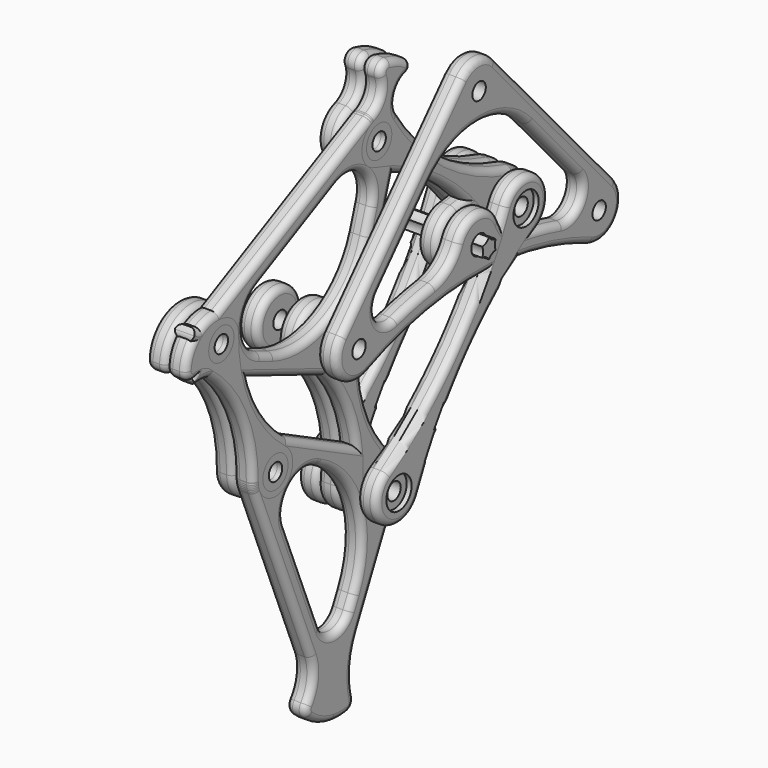
from build123d import *

# Parameters (mm, degrees)
F9_START        = -20
F4_R            = 14.25
F4_R_2          = 4.25
F9_DEPTH        = 10
F10_DEPTH       = 25
F5_R            = 4.25
F11_DEPTH       = 10
F12_DEPTH       = 10
F6_R            = 4.25
F13_DEPTH       = 10
F14_START       = -10
F7_R            = 4.25
F14_DEPTH       = 10
F15_START       = 10
F8_R            = 4.25
F15_DEPTH       = 10
F16_F1_R        = 3.3333333333
F16_F2_R        = 3.3333333333
F16_2_T1_DEPTH  = 111.6
F16_2_T3_DEPTH  = 23.6921609305
F16_2_T5_DEPTH  = 83
F16_2_T7_DEPTH  = 9.0519604966
F16_2_T9_DEPTH  = 55.2336790395
F16_2_T11_DEPTH = 12.4143797947
F16_2_T13_DEPTH = 80.2
F16_2_T16_ANGLE = 132.0850519137
F16_2_T18_ANGLE = 201.4453377433
F16_2_T20_ANGLE = 201.4453377433
F16_2_T22_ANGLE = 100.7027482307
F16_2_T24_ANGLE = 100.7027482307
F16_2_T26_ANGLE = 54.6379434109
F16_2_T28_ANGLE = 54.6379434109
F16_2_T30_ANGLE = 134.1832559662
F16_2_T32_ANGLE = 134.1832559662
F16_2_T34_ANGLE = 93.7316921202
F16_2_T36_ANGLE = 134.1832559662
F16_2_T38_ANGLE = 134.1832559662
F16_2_T40_ANGLE = 93.7316921202
F16_2_T42_ANGLE = 132.0850519137
F16_2_T44_ANGLE = 93.7316921202
F16_2_T46_ANGLE = 93.7316921202
F16_3_F1_R      = 3.3333333333
F16_4_F1_R      = 3.3333333333
F16_4_F2_R      = 3.3333333333
F16_4_F3_R      = 3.3333333333
F16_4_F4_R      = 3.3333333333
F16_5_F1_R      = 3.3333333333
F16_5_F2_R      = 3.3333333333
F16_6_F1_R      = 3.3333333333
F16_7_F1_R      = 3.3333333333
F16_8_F1_R      = 3.3333333333
F16_8_F2_R      = 3.3333333333
F16_9_F1_R      = 3.3333333333
F16_9_F2_R      = 3.3333333333
F17_R           = 8
F17_R_2         = 4.25
F18_DEPTH       = 2.5
F19_R           = 8
F19_R_2         = 4.25
F20_DEPTH       = 2.5
F21_R           = 8
F21_R_2         = 4.25
F22_DEPTH       = 2.5
F23_R           = 8
F23_R_2         = 4.25
F24_DEPTH       = 2.5


# Not quite as in the source:
# - a fillet or chamfer that OpenCascade refuses, or shapes differently, is made with other operations: its cross-section is extruded or revolved along the edge and cut away or added


with BuildPart() as f9:
    # F4 (on Right) → F9 (new body)
    with BuildSketch(Plane.YZ.offset(F9_START)):
        with Locations((-76, -15.6)):
            Circle(F4_R)
        with Locations((-76, -15.6)):
            Circle(F4_R_2, mode=Mode.SUBTRACT)
    extrude(amount=-F9_DEPTH)

    # F16: fillet of radius 3.3333333333 on 3 edges, made by hand

    # F16_f1
    f16_f1_edges = [f9.edges().sort_by_distance(p)[0] for p in [
        (-20, -90.25, -15.6),
    ]]
    fillet(f16_f1_edges, radius=F16_F1_R)

    # F16_f2
    f16_f2_edges = [f9.edges().sort_by_distance(p)[0] for p in [
        (-30, -90.25, -15.6),
    ]]
    fillet(f16_f2_edges, radius=F16_F2_R)


with BuildPart() as f10:
    # F3 (on Right) → F10 (new body, symmetric)
    with BuildSketch(Plane.YZ):
        with BuildLine():
            ThreePointArc((-4.2835398746, 2.4731028997), (-3.6961524227, 0), (-4.2835398746, -2.4731028997))
            ThreePointArc((-4.2835398746, -2.4731028997), (-1.8480762114, -3.2009618943), (0, -4.9462057994))
            ThreePointArc((0, -4.9462057994), (1.8480762114, -3.2009618943), (4.2835398746, -2.4731028997))
            ThreePointArc((4.2835398746, -2.4731028997), (3.6961524227, 0), (4.2835398746, 2.4731028997))
            ThreePointArc((4.2835398746, 2.4731028997), (1.8480762114, 3.2009618943), (0, 4.9462057994))
            ThreePointArc((0, 4.9462057994), (-1.8480762114, 3.2009618943), (-4.2835398746, 2.4731028997))
        make_face()
    extrude(amount=F10_DEPTH, both=True)


with BuildPart() as f11:
    # F5 (on Right) → F11 (new body)
    with BuildSketch(Plane.YZ):
        with BuildLine():
            Line((-57.1063179985, 76.2227923438), (-157.0028723597, 26.471024267))
            ThreePointArc((-157.0028723597, 26.471024267), (-162.7660308401, 21.2166273966), (-164.900160038, 13.7154158472))
            ThreePointArc((-164.900160038, 13.7154158472), (-162.4248725051, 5.6892931022), (-155.8589465196, 0.4515158405))
            Line((-155.8589465196, 0.4515158405), (-81.2087864816, -28.8639000068))
            ThreePointArc((-81.2087864816, -28.8639000068), (-69.8818983437, -28.469783686), (-62.4252123986, -19.9344713145))
            Line((-62.4252123986, -19.9344713145), (-37.1788180755, 59.1327126096))
            ThreePointArc((-37.1788180755, 59.1327126096), (-41.4768983317, 74.2840781563), (-57.1063179985, 76.2227923438))
        make_face()
        with Locations((-76, -15.6)):
            Circle(F5_R, mode=Mode.SUBTRACT)
        with Locations((-150.650160038, 13.7154158472)):
            Circle(F5_R, mode=Mode.SUBTRACT)
        with BuildLine():
            ThreePointArc((-125.7090220308, -0.6450333714), (-136.4139116441, 14.3413005541), (-127.0655051666, 30.2092608039))
            Line((-127.0655051666, 30.2092608039), (-77.6241591027, 54.8326764813))
            ThreePointArc((-77.6241591027, 54.8326764813), (-60.030313022, 52.6502896918), (-55.192016778, 35.5945832725))
            Line((-55.192016778, 35.5945832725), (-58.9681412066, 23.7684380854))
            ThreePointArc((-58.9681412066, 23.7684380854), (-82.1181016563, -2.730216314), (-117.2834571963, -3.9537863164))
            Line((-117.2834571963, -3.9537863164), (-125.7090220308, -0.6450333714))
        make_face(mode=Mode.SUBTRACT)
        with Locations((-50.7536056769, 63.4671839241)):
            Circle(F5_R, mode=Mode.SUBTRACT)
        with BuildLine():
            ThreePointArc((-164.900160038, 13.7154158472), (-162.7660308401, 21.2166273966), (-157.0028723597, 26.471024267))
            ThreePointArc((-157.0028723597, 26.471024267), (-161.4609160942, 25.4223284212), (-165.9189598286, 26.471024267))
            ThreePointArc((-165.9189598286, 26.471024267), (-167.5662735959, 24.188567011), (-168.8749908257, 21.6964769273))
            ThreePointArc((-168.8749908257, 21.6964769273), (-165.9488558838, 18.1734595817), (-164.900160038, 13.7154158472))
        make_face()
        with BuildLine():
            ThreePointArc((-155.8589465196, 0.4515158405), (-162.4248725051, 5.6892931022), (-164.900160038, 13.7154158472))
            ThreePointArc((-164.900160038, 13.7154158472), (-165.9488558838, 9.2573721128), (-168.8749908257, 5.7343547672))
            ThreePointArc((-168.8749908257, 5.7343547672), (-167.7693516826, 3.5776118128), (-166.4096773207, 1.5713058254))
            ThreePointArc((-166.4096773207, 1.5713058254), (-161.0587017415, 1.7238146329), (-155.8589465196, 0.4515158405))
        make_face()
    extrude(amount=F11_DEPTH)

    # F16#2: fillet of radius 3.3333333333 on 28 edges, made by hand

    # F16_2_s2 → F16_2_t1 (cut)
    with BuildSketch(Plane(origin=(0, -15.3399823815, -7.6398155134), x_dir=(1, 0, 0), z_dir=(0, -0.8951304154, -0.4458043734))):
        with BuildLine():
            ThreePointArc((3.3333333333, 93.6875860907), (0.9763107294, 92.7112753613), (0, 90.3542527573))
            Line((0, 90.3542527573), (0, 93.6875860907))
            Line((0, 93.6875860907), (3.3333333333, 93.6875860907))
        make_face()
        with BuildLine():
            ThreePointArc((6.6666666667, 93.6875860907), (9.0236892706, 92.7112753613), (10, 90.3542527573))
            Line((10, 90.3542527573), (10, 93.6875860907))
            Line((10, 93.6875860907), (6.6666666667, 93.6875860907))
        make_face()
    extrude(amount=F16_2_T1_DEPTH, mode=Mode.SUBTRACT)

    # F16_2_s4 → F16_2_t3 (cut)
    with BuildSketch(Plane.YZ.offset(-6.8460804653)):
        with BuildLine():
            ThreePointArc((-167.6064610002, 24.1233767851), (-168.0886966243, 22.1185143512), (-167.2992446495, 20.2135759911))
            ThreePointArc((-167.2992446495, 20.2135759911), (-168.0468911695, 20.9977716348), (-168.8749908257, 21.6964769273))
            ThreePointArc((-168.8749908257, 21.6964769273), (-168.2825299449, 22.9317776388), (-167.6064610002, 24.1233767851))
        make_face()
        with BuildLine():
            ThreePointArc((-167.2992446495, 7.2172557033), (-168.0886966243, 5.3123173433), (-167.6064610002, 3.3074549094))
            ThreePointArc((-167.6064610002, 3.3074549094), (-168.2825299449, 4.4990540557), (-168.8749908257, 5.7343547672))
            ThreePointArc((-168.8749908257, 5.7343547672), (-168.0468911695, 6.4330600597), (-167.2992446495, 7.2172557033))
        make_face()
    extrude(amount=F16_2_T3_DEPTH, mode=Mode.SUBTRACT)

    # F16_2_s6 → F16_2_t5 (cut)
    with BuildSketch(Plane(origin=(0, -11.5518984951, -36.1784764705), x_dir=(1, 0, 0), z_dir=(0, 0.3041734256, 0.9526166738))):
        with BuildLine():
            ThreePointArc((3.3333333333, -53.4037617685), (0.9763107294, -54.3800724979), (0, -56.7370951019))
            Line((0, -56.7370951019), (0, -53.4037617685))
            Line((0, -53.4037617685), (3.3333333333, -53.4037617685))
        make_face()
        with BuildLine():
            ThreePointArc((6.6666666667, -53.4037617685), (9.0236892706, -54.3800724979), (10, -56.7370951019))
            Line((10, -56.7370951019), (10, -53.4037617685))
            Line((10, -53.4037617685), (6.6666666667, -53.4037617685))
        make_face()
    extrude(amount=F16_2_T5_DEPTH, mode=Mode.SUBTRACT)

    # F16_2_s8 → F16_2_t7 (cut)
    with BuildSketch(Plane(origin=(0, -100.2678414461, 39.3755816009), x_dir=(1, 0, 0), z_dir=(0, -0.9308000005, 0.3655288759))):
        with BuildLine():
            ThreePointArc((3.3333333333, -46.5506745758), (0.9763107294, -47.5269853052), (0, -49.8840079092))
            Line((0, -49.8840079092), (0, -46.5506745758))
            Line((0, -46.5506745758), (3.3333333333, -46.5506745758))
        make_face()
        with BuildLine():
            ThreePointArc((6.6666666667, -46.5506745758), (9.0236892706, -47.5269853052), (10, -49.8840079092))
            Line((10, -49.8840079092), (10, -46.5506745758))
            Line((10, -46.5506745758), (6.6666666667, -46.5506745758))
        make_face()
    extrude(amount=F16_2_T7_DEPTH, mode=Mode.SUBTRACT)

    # F16_2_s10 → F16_2_t9 (cut)
    with BuildSketch(Plane(origin=(0, -89.7572132841, -44.7020428992), x_dir=(1, 0, 0), z_dir=(0, 0.8951304154, 0.4458043734))):
        with BuildLine():
            ThreePointArc((3.3333333333, -83.6875860907), (0.9763107294, -84.66389682), (0, -87.020919424))
            Line((0, -87.020919424), (0, -83.6875860907))
            Line((0, -83.6875860907), (3.3333333333, -83.6875860907))
        make_face()
        with BuildLine():
            ThreePointArc((6.6666666667, -83.6875860907), (9.0236892706, -84.66389682), (10, -87.020919424))
            Line((10, -87.020919424), (10, -83.6875860907))
            Line((10, -83.6875860907), (6.6666666667, -83.6875860907))
        make_face()
    extrude(amount=F16_2_T9_DEPTH, mode=Mode.SUBTRACT)

    # F16_2_s12 → F16_2_t11 (cut)
    with BuildSketch(Plane(origin=(0, 5.2074638633, 16.3088438607), x_dir=(1, 0, 0), z_dir=(0, -0.3041734256, -0.9526166738))):
        with BuildLine():
            ThreePointArc((3.3333333333, 63.4037617685), (0.9763107294, 62.4274510392), (0, 60.0704284352))
            Line((0, 60.0704284352), (0, 63.4037617685))
            Line((0, 63.4037617685), (3.3333333333, 63.4037617685))
        make_face()
        with BuildLine():
            ThreePointArc((6.6666666667, 63.4037617685), (9.0236892706, 62.4274510392), (10, 60.0704284352))
            Line((10, 60.0704284352), (10, 63.4037617685))
            Line((10, 63.4037617685), (6.6666666667, 63.4037617685))
        make_face()
    extrude(amount=F16_2_T11_DEPTH, mode=Mode.SUBTRACT)

    # F16_2_s14 → F16_2_t13 (cut)
    with BuildSketch(Plane(origin=(0, -135.1880420105, 53.0888837625), x_dir=(1, 0, 0), z_dir=(0, 0.9308000005, -0.3655288759))):
        with BuildLine():
            ThreePointArc((6.6666666667, 56.5506745758), (9.0236892706, 55.5743638465), (10, 53.2173412425))
            Line((10, 53.2173412425), (10, 56.5506745758))
            Line((10, 56.5506745758), (6.6666666667, 56.5506745758))
        make_face()
        with BuildLine():
            ThreePointArc((3.3333333333, 56.5506745758), (0.9763107294, 55.5743638465), (0, 53.2173412425))
            Line((0, 53.2173412425), (0, 56.5506745758))
            Line((0, 56.5506745758), (3.3333333333, 56.5506745758))
        make_face()
    extrude(amount=F16_2_T13_DEPTH, mode=Mode.SUBTRACT)

    # F16_2_s15 → F16_2_t16 (revolve, cut)
    with BuildSketch(Plane(origin=(0, -108.6934062806, 42.6843345459), x_dir=(1, 0, 0), z_dir=(0, 0.9308000005, -0.3655288759))):
        with BuildLine():
            ThreePointArc((6.6666666667, 46.5506745758), (9.0236892706, 47.5269853052), (10, 49.8840079092))
            Line((10, 49.8840079092), (10, 46.5506745758))
            Line((10, 46.5506745758), (6.6666666667, 46.5506745758))
        make_face()
    revolve(axis=Axis((10, -119.5323707365, 15.0834833251), (-1, 0, 0)), revolution_arc=F16_2_T16_ANGLE, mode=Mode.SUBTRACT)

    # F16_2_s17 → F16_2_t18 (revolve, cut)
    with BuildSketch(Plane(origin=(0, -166.3384411937, -31.4981407109), x_dir=(1, 0, 0), z_dir=(0, -0.9825392613, -0.1860553681))):
        with BuildLine():
            ThreePointArc((3.3333333333, 56.0170482127), (0.9763107294, 56.9933589421), (0, 59.350381546))
            Line((0, 59.350381546), (0, 56.0170482127))
            Line((0, 56.0170482127), (3.3333333333, 56.0170482127))
        make_face()
    revolve(axis=Axis((0, -174.900160038, 13.7154158472), (-1, 0, 0)), revolution_arc=F16_2_T18_ANGLE, mode=Mode.SUBTRACT)

    # F16_2_s19 → F16_2_t20 (revolve, cut)
    with BuildSketch(Plane(origin=(0, -166.3384411937, -31.4981407109), x_dir=(1, 0, 0), z_dir=(0, -0.9825392613, -0.1860553681))):
        with BuildLine():
            ThreePointArc((6.6666666667, 56.0170482127), (9.0236892706, 56.9933589421), (10, 59.350381546))
            Line((10, 59.350381546), (10, 56.0170482127))
            Line((10, 56.0170482127), (6.6666666667, 56.0170482127))
        make_face()
    revolve(axis=Axis((10, -174.900160038, 13.7154158472), (-1, 0, 0)), revolution_arc=F16_2_T20_ANGLE, mode=Mode.SUBTRACT)

    # F16_2_s21 → F16_2_t22 (revolve, cut)
    with BuildSketch(Plane(origin=(0, -115.2365367426, -57.3915835903), x_dir=(1, 0, 0), z_dir=(0, 0.8951304154, 0.4458043734))):
        with BuildLine():
            ThreePointArc((3.3333333333, -93.6875860907), (0.9763107294, -92.7112753613), (0, -90.3542527573))
            Line((0, -90.3542527573), (0, -93.6875860907))
            Line((0, -93.6875860907), (3.3333333333, -93.6875860907))
        make_face()
    revolve(axis=Axis((0, -161.4609160942, 35.4223284212), (-1, 0, 0)), revolution_arc=F16_2_T22_ANGLE, mode=Mode.SUBTRACT)

    # F16_2_s23 → F16_2_t24 (revolve, cut)
    with BuildSketch(Plane(origin=(0, -115.2365367426, -57.3915835903), x_dir=(1, 0, 0), z_dir=(0, 0.8951304154, 0.4458043734))):
        with BuildLine():
            ThreePointArc((6.6666666667, -93.6875860907), (9.0236892706, -92.7112753613), (10, -90.3542527573))
            Line((10, -90.3542527573), (10, -93.6875860907))
            Line((10, -93.6875860907), (6.6666666667, -93.6875860907))
        make_face()
    revolve(axis=Axis((10, -161.4609160942, 35.4223284212), (-1, 0, 0)), revolution_arc=F16_2_T24_ANGLE, mode=Mode.SUBTRACT)

    # F16_2_s25 → F16_2_t26 (revolve, cut)
    with BuildSketch(Plane(origin=(0, -122.5752098671, -80.2042759428), x_dir=(1, 0, 0), z_dir=(0, -0.8367852502, -0.5475312274))):
        with BuildLine():
            ThreePointArc((3.3333333333, 94.1406373476), (0.9763107294, 95.116948077), (0, 97.4739706809))
            Line((0, 97.4739706809), (0, 94.1406373476))
            Line((0, 94.1406373476), (3.3333333333, 94.1406373476))
        make_face()
    revolve(axis=Axis((0, -163.1695240376, -18.164484169), (-1, 0, 0)), revolution_arc=F16_2_T26_ANGLE, mode=Mode.SUBTRACT)

    # F16_2_s27 → F16_2_t28 (revolve, cut)
    with BuildSketch(Plane(origin=(0, -122.5752098671, -80.2042759428), x_dir=(1, 0, 0), z_dir=(0, -0.8367852502, -0.5475312274))):
        with BuildLine():
            ThreePointArc((6.6666666667, 94.1406373476), (9.0236892706, 95.116948077), (10, 97.4739706809))
            Line((10, 97.4739706809), (10, 94.1406373476))
            Line((10, 94.1406373476), (6.6666666667, 94.1406373476))
        make_face()
    revolve(axis=Axis((10, -163.1695240376, -18.164484169), (-1, 0, 0)), revolution_arc=F16_2_T28_ANGLE, mode=Mode.SUBTRACT)

    # F16_2_s29 → F16_2_t30 (revolve, cut)
    with BuildSketch(Plane(origin=(0, 13.694495828, 42.8887074536), x_dir=(1, 0, 0), z_dir=(0, -0.3041734256, -0.9526166738))):
        with BuildLine():
            ThreePointArc((3.3333333333, 53.4037617685), (0.9763107294, 54.3800724979), (0, 56.7370951019))
            Line((0, 56.7370951019), (0, 53.4037617685))
            Line((0, 53.4037617685), (3.3333333333, 53.4037617685))
        make_face()
    revolve(axis=Axis((0, -50.7536056769, 63.4671839241), (1, 0, 0)), revolution_arc=F16_2_T30_ANGLE, mode=Mode.SUBTRACT)

    # F16_2_s31 → F16_2_t32 (revolve, cut)
    with BuildSketch(Plane(origin=(0, 13.694495828, 42.8887074536), x_dir=(1, 0, 0), z_dir=(0, -0.3041734256, -0.9526166738))):
        with BuildLine():
            ThreePointArc((6.6666666667, 53.4037617685), (9.0236892706, 54.3800724979), (10, 56.7370951019))
            Line((10, 56.7370951019), (10, 53.4037617685))
            Line((10, 53.4037617685), (6.6666666667, 53.4037617685))
        make_face()
    revolve(axis=Axis((10, -50.7536056769, 63.4671839241), (1, 0, 0)), revolution_arc=F16_2_T32_ANGLE, mode=Mode.SUBTRACT)

    # F16_2_s33 → F16_2_t34 (revolve, cut)
    with BuildSketch(Plane(origin=(0, 1.4313394348, 4.4826986736), x_dir=(1, 0, 0), z_dir=(0, 0.3041734256, 0.9526166738))):
        with BuildLine():
            ThreePointArc((3.3333333333, -63.4037617685), (0.9763107294, -62.4274510392), (0, -60.0704284352))
            Line((0, -60.0704284352), (0, -63.4037617685))
            Line((0, -63.4037617685), (3.3333333333, -63.4037617685))
        make_face()
    revolve(axis=Axis((0, -101.1123053029, 37.2251989359), (-1, 0, 0)), revolution_arc=F16_2_T34_ANGLE, mode=Mode.SUBTRACT)

    # F16_2_s35 → F16_2_t36 (revolve, cut)
    with BuildSketch(Plane(origin=(0, -40.3158672201, -20.0786272217), x_dir=(1, 0, 0), z_dir=(0, -0.8951304154, -0.4458043734))):
        with BuildLine():
            ThreePointArc((3.3333333333, 83.6875860907), (0.9763107294, 84.66389682), (0, 87.020919424))
            Line((0, 87.020919424), (0, 83.6875860907))
            Line((0, 83.6875860907), (3.3333333333, 83.6875860907))
        make_face()
    revolve(axis=Axis((0, -70.4729887352, 40.4738444846), (-1, 0, 0)), revolution_arc=F16_2_T36_ANGLE, mode=Mode.SUBTRACT)

    # F16_2_s37 → F16_2_t38 (revolve, cut)
    with BuildSketch(Plane(origin=(0, -40.3158672201, -20.0786272217), x_dir=(1, 0, 0), z_dir=(0, -0.8951304154, -0.4458043734))):
        with BuildLine():
            ThreePointArc((6.6666666667, 83.6875860907), (9.0236892706, 84.66389682), (10, 87.020919424))
            Line((10, 87.020919424), (10, 83.6875860907))
            Line((10, 83.6875860907), (6.6666666667, 83.6875860907))
        make_face()
    revolve(axis=Axis((10, -70.4729887352, 40.4738444846), (-1, 0, 0)), revolution_arc=F16_2_T38_ANGLE, mode=Mode.SUBTRACT)

    # F16_2_s39 → F16_2_t40 (revolve, cut)
    with BuildSketch(Plane(origin=(0, 1.4313394348, 4.4826986736), x_dir=(1, 0, 0), z_dir=(0, 0.3041734256, 0.9526166738))):
        with BuildLine():
            ThreePointArc((6.6666666667, -63.4037617685), (9.0236892706, -62.4274510392), (10, -60.0704284352))
            Line((10, -60.0704284352), (10, -63.4037617685))
            Line((10, -63.4037617685), (6.6666666667, -63.4037617685))
        make_face()
    revolve(axis=Axis((10, -101.1123053029, 37.2251989359), (-1, 0, 0)), revolution_arc=F16_2_T40_ANGLE, mode=Mode.SUBTRACT)

    # F16_2_s41 → F16_2_t42 (revolve, cut)
    with BuildSketch(Plane(origin=(0, -108.6934062806, 42.6843345459), x_dir=(1, 0, 0), z_dir=(0, 0.9308000005, -0.3655288759))):
        with BuildLine():
            ThreePointArc((3.3333333333, 46.5506745758), (0.9763107294, 47.5269853052), (0, 49.8840079092))
            Line((0, 49.8840079092), (0, 46.5506745758))
            Line((0, 46.5506745758), (3.3333333333, 46.5506745758))
        make_face()
    revolve(axis=Axis((0, -119.5323707365, 15.0834833251), (-1, 0, 0)), revolution_arc=F16_2_T42_ANGLE, mode=Mode.SUBTRACT)

    # F16_2_s43 → F16_2_t44 (revolve, cut)
    with BuildSketch(Plane(origin=(0, -60.5378819724, 23.7734679153), x_dir=(1, 0, 0), z_dir=(0, -0.9308000005, 0.3655288759))):
        with BuildLine():
            ThreePointArc((6.6666666667, -56.5506745758), (9.0236892706, -55.5743638465), (10, -53.2173412425))
            Line((10, -53.2173412425), (10, -56.5506745758))
            Line((10, -56.5506745758), (6.6666666667, -56.5506745758))
        make_face()
    revolve(axis=Axis((10, -76, -15.6), (1, 0, 0)), revolution_arc=F16_2_T44_ANGLE, mode=Mode.SUBTRACT)

    # F16_2_s45 → F16_2_t46 (revolve, cut)
    with BuildSketch(Plane(origin=(0, -60.5378819724, 23.7734679153), x_dir=(1, 0, 0), z_dir=(0, -0.9308000005, 0.3655288759))):
        with BuildLine():
            ThreePointArc((3.3333333333, -56.5506745758), (0.9763107294, -55.5743638465), (0, -53.2173412425))
            Line((0, -53.2173412425), (0, -56.5506745758))
            Line((0, -56.5506745758), (3.3333333333, -56.5506745758))
        make_face()
    revolve(axis=Axis((0, -76, -15.6), (1, 0, 0)), revolution_arc=F16_2_T46_ANGLE, mode=Mode.SUBTRACT)


with BuildPart() as f11b:
    # F5 (on Right) → F11, piece 2 (new body)
    with BuildSketch(Plane.YZ):
        with BuildLine():
            ThreePointArc((-110.0171751391, -44.4920792731), (-126.0763947693, -46.799791208), (-129.5669264658, -62.6440412054))
            Line((-129.5669264658, -62.6440412054), (-93.817508921, -149.9170955083))
            Line((-93.817508921, -149.9170955083), (-80.052473801, -183.5209061437))
            Line((-80.052473801, -183.5209061437), (-63.817508921, -149.9170955083))
            Line((-63.817508921, -149.9170955083), (-37.8736864923, -96.2174846691))
            ThreePointArc((-37.8736864923, -96.2174846691), (-37.218611188, -85.4153913463), (-44.3415008039, -77.2680735467))
            Line((-44.3415008039, -77.2680735467), (-110.0171751391, -44.4920792731))
        make_face()
        with BuildLine():
            ThreePointArc((-69.5436558742, -138.7818275874), (-78.8542275315, -144.4269408432), (-87.8015966731, -138.2222141207))
            Line((-87.8015966731, -138.2222141207), (-110.1854942304, -83.5776564974))
            ThreePointArc((-110.1854942304, -83.5776564974), (-106.6843293072, -67.6851400706), (-90.5761883844, -65.3703981397))
            Line((-90.5761883844, -65.3703981397), (-89.1351981073, -66.0895363829))
            ThreePointArc((-89.1351981073, -66.0895363829), (-64.1907642182, -94.6215284794), (-66.4848447814, -132.4505722079))
            Line((-66.4848447814, -132.4505722079), (-69.5436558742, -138.7818275874))
        make_face(mode=Mode.SUBTRACT)
        with Locations((-116.3803620382, -57.2424656393)):
            Circle(F5_R, mode=Mode.SUBTRACT)
        with Locations((-50.7046877031, -90.0184599129)):
            Circle(F5_R, mode=Mode.SUBTRACT)
        with BuildLine():
            Line((-80.052473801, -183.5209061437), (-93.817508921, -149.9170955083))
            ThreePointArc((-93.817508921, -149.9170955083), (-92.4766246704, -159.9565618129), (-96.2262873625, -169.3655407133))
            ThreePointArc((-96.2262873625, -169.3655407133), (-97.1781166541, -172.8165666329), (-95.5788811028, -176.0193786083))
            ThreePointArc((-95.5788811028, -176.0193786083), (-88.3662640694, -180.9097278853), (-80.052473801, -183.5209061437))
        make_face()
        with BuildLine():
            Line((-63.817508921, -149.9170955083), (-80.052473801, -183.5209061437))
            ThreePointArc((-80.052473801, -183.5209061437), (-75.315298055, -183.8972810119), (-70.5781223089, -183.5209061437))
            ThreePointArc((-70.5781223089, -183.5209061437), (-67.1842215616, -181.3220496315), (-66.5268751351, -177.331883229))
            ThreePointArc((-66.5268751351, -177.331883229), (-67.6067408069, -163.3838862214), (-63.817508921, -149.9170955083))
        make_face()
    extrude(amount=F11_DEPTH)

    # F16#4: fillet of radius 3.3333333333 on 31 edges, made by hand

    # F16_4_f1
    f16_4_f1_edges = [f11b.edges().sort_by_distance(p)[0] for p in [
        (0, -37.218611188, -85.4153913463),
        (0, -77.1793379715, -60.8800764099),
        (0, -126.0763947693, -46.799791208),
        (0, -111.6922176934, -106.2805683569),
        (0, -92.4766246704, -159.9565618129),
        (0, -97.1781166541, -172.8165666329),
        (0, -83.9371052765, -182.6316583365),
        (0, -67.1842215616, -181.3220496315),
        (0, -67.6067408069, -163.3838862214),
        (0, -50.8455977066, -123.0672900887),
    ]]
    fillet(f16_4_f1_edges, radius=F16_4_F1_R)

    # F16_4_f2
    f16_4_f2_edges = [f11b.edges().sort_by_distance(p)[0] for p in [
        (10, -37.218611188, -85.4153913463),
        (10, -77.1793379715, -60.8800764099),
        (10, -126.0763947693, -46.799791208),
        (10, -111.6922176934, -106.2805683569),
        (10, -92.4766246704, -159.9565618129),
        (10, -97.1781166541, -172.8165666329),
        (10, -83.9371052765, -182.6316583365),
        (10, -67.1842215616, -181.3220496315),
        (10, -67.6067408069, -163.3838862214),
        (10, -50.8455977066, -123.0672900887),
    ]]
    fillet(f16_4_f2_edges, radius=F16_4_F2_R)

    # F16_4_f3
    f16_4_f3_edges = [f11b.edges().sort_by_distance(p)[0] for p in [
        (0, -78.8542275315, -144.4269408432),
        (0, -98.9935454517, -110.899935309),
        (0, -106.6843293072, -67.6851400706),
        (0, -89.8556932459, -65.7299672613),
        (0, -64.1907642182, -94.6215284794),
        (0, -68.0142503278, -135.6161998976),
    ]]
    fillet(f16_4_f3_edges, radius=F16_4_F3_R)

    # F16_4_f4
    f16_4_f4_edges = [f11b.edges().sort_by_distance(p)[0] for p in [
        (10, -78.8542275315, -144.4269408432),
        (10, -98.9935454517, -110.899935309),
        (10, -106.6843293072, -67.6851400706),
        (10, -89.8556932459, -65.7299672613),
        (10, -64.1907642182, -94.6215284794),
        (10, -68.0142503278, -135.6161998976),
    ]]
    fillet(f16_4_f4_edges, radius=F16_4_F4_R)


with BuildPart() as f12:
    # F5 (on Right) → F12 (new body)
    with BuildSketch(Plane.YZ):
        with BuildLine():
            Line((27.7700369033, 18.2177811599), (-1.9482561751, 14.1161892123))
            ThreePointArc((-1.9482561751, 14.1161892123), (-14.1161892123, -1.9482561751), (1.9482561751, -14.1161892123))
            Line((1.9482561751, -14.1161892123), (31.6665492535, -10.0145972646))
            ThreePointArc((31.6665492535, -10.0145972646), (43.8344822907, 6.0498481227), (27.7700369033, 18.2177811599))
        make_face()
        with BuildLine():
            ThreePointArc((-5.1961524227, -3), (-4.1961524227, 0), (-5.1961524227, 3))
            ThreePointArc((-5.1961524227, 3), (-2.0980762114, 3.6339745962), (0, 6))
            ThreePointArc((0, 6), (2.0980762114, 3.6339745962), (5.1961524227, 3))
            ThreePointArc((5.1961524227, 3), (4.1961524227, 0), (5.1961524227, -3))
            ThreePointArc((5.1961524227, -3), (2.0980762114, -3.6339745962), (0, -6))
            ThreePointArc((0, -6), (-2.0980762114, -3.6339745962), (-5.1961524227, -3))
        make_face(mode=Mode.SUBTRACT)
        with Locations((29.7182930784, 4.1015919476)):
            Circle(F5_R, mode=Mode.SUBTRACT)
    extrude(amount=F12_DEPTH)

    # F16#5: fillet of radius 3.3333333333 on 10 edges, made by hand

    # F16_5_f1
    f16_5_f1_edges = [f12.edges().sort_by_distance(p)[0] for p in [
        (0, 43.8344822907, 6.0498481227),
        (0, 12.9108903641, 16.1669851861),
        (0, -14.1161892123, -1.9482561751),
        (0, 16.8074027143, -12.0653932384),
    ]]
    fillet(f16_5_f1_edges, radius=F16_5_F1_R)

    # F16_5_f2
    f16_5_f2_edges = [f12.edges().sort_by_distance(p)[0] for p in [
        (10, 43.8344822907, 6.0498481227),
        (10, 12.9108903641, 16.1669851861),
        (10, -14.1161892123, -1.9482561751),
        (10, 16.8074027143, -12.0653932384),
    ]]
    fillet(f16_5_f2_edges, radius=F16_5_F2_R)


with BuildPart() as f13:
    # F6 (on Right) → F13 (new body)
    with BuildSketch(Plane.YZ):
        with BuildLine():
            ThreePointArc((-107.647019446, -45.9823045762), (-129.0128573905, -19.5890453275), (-136.4010647178, 13.5548463771))
            ThreePointArc((-136.4010647178, 13.5548463771), (-138.5375973787, 21.22196804), (-144.4528932678, 26.547266243))
            ThreePointArc((-144.4528932678, 26.547266243), (-162.7627226974, 21.22196804), (-159.3835026302, 2.4552547841))
            ThreePointArc((-159.3835026302, 2.4552547841), (-138.0176646858, -23.9380044645), (-130.6294573585, -57.0818961691))
            ThreePointArc((-130.6294573585, -57.0818961691), (-110.183095268, -70.074316035), (-107.647019446, -45.9823045762))
        make_face()
        with Locations((-116.3803620382, -57.2424656393)):
            Circle(F6_R, mode=Mode.SUBTRACT)
        with Locations((-150.650160038, 13.7154158472)):
            Circle(F6_R, mode=Mode.SUBTRACT)
        with BuildLine():
            ThreePointArc((-159.3835026302, 2.4552547841), (-162.7627226974, 21.22196804), (-144.4528932678, 26.547266243))
            ThreePointArc((-144.4528932678, 26.547266243), (-163.3345833201, 25.7507510935), (-173.1233705354, 9.5849755023))
            ThreePointArc((-173.1233705354, 9.5849755023), (-171.441695893, 5.5769199267), (-167.2575418908, 4.3998921504))
            ThreePointArc((-167.2575418908, 4.3998921504), (-163.1145199282, 4.2616983694), (-159.3835026302, 2.4552547841))
        make_face()
    extrude(amount=-F13_DEPTH)

    # F16#3: fillet of radius 3.3333333333 on 14 edges, made by hand

    # F16_3_f1
    f16_3_f1_edges = [f13.edges().sort_by_distance(p)[0] for p in [
        (0, -138.5375973787, 21.22196804),
        (0, -163.3345833201, 25.7507510935),
        (-10, -163.3345833201, 25.7507510935),
        (-10, -129.0128573905, -19.5890453275),
        (-10, -138.5375973787, 21.22196804),
        (0, -171.441695893, 5.5769199267),
        (-10, -171.441695893, 5.5769199267),
        (0, -163.1145199282, 4.2616983694),
        (-10, -163.1145199282, 4.2616983694),
        (0, -138.0176646858, -23.9380044645),
        (-10, -138.0176646858, -23.9380044645),
        (-10, -110.183095268, -70.074316035),
        (0, -110.183095268, -70.074316035),
        (0, -129.0128573905, -19.5890453275),
    ]]
    fillet(f16_3_f1_edges, radius=F16_3_F1_R)

    # F17 (on face) → F18 (cut)
    with BuildSketch(Plane(origin=(-10, 0, 0), x_dir=(0, -1, 0), z_dir=(-1, 0, 0))):
        with Locations((150.650160038, 13.7154158472)):
            Circle(F17_R)
        with Locations((150.650160038, 13.7154158472)):
            Circle(F17_R_2, mode=Mode.SUBTRACT)
        with Locations((116.3803620382, -57.2424656393)):
            Circle(F17_R)
        with Locations((116.3803620382, -57.2424656393)):
            Circle(F17_R_2, mode=Mode.SUBTRACT)
    extrude(amount=-F18_DEPTH, mode=Mode.SUBTRACT)


with BuildPart() as f13b:
    # F6 (on Right) → F13, piece 2 (new body)
    with BuildSketch(Plane.YZ):
        with BuildLine():
            ThreePointArc((-40.6746670307, -79.8961486495), (-58.6183451293, -51.2001133981), (-61.879021089, -17.5132314536))
            ThreePointArc((-61.879021089, -17.5132314536), (-80.5859821912, -2.1081036418), (-86.0300206724, -25.7223112633))
            ThreePointArc((-86.0300206724, -25.7223112633), (-68.0863425737, -54.4183465148), (-64.8256666141, -88.1052284593))
            ThreePointArc((-64.8256666141, -88.1052284593), (-46.1187055118, -103.5103562711), (-40.6746670307, -79.8961486495))
        make_face()
        with Locations((-76, -15.6)):
            Circle(F6_R, mode=Mode.SUBTRACT)
        with Locations((-50.7046877031, -90.0184599129)):
            Circle(F6_R, mode=Mode.SUBTRACT)
    extrude(amount=-F13_DEPTH)

    # F16#6: fillet of radius 3.3333333333 on 8 edges, made by hand

    # F16_6_f1
    f16_6_f1_edges = [f13b.edges().sort_by_distance(p)[0] for p in [
        (0, -80.5859821912, -2.1081036418),
        (-10, -80.5859821912, -2.1081036418),
        (0, -58.6183451293, -51.2001133981),
        (-10, -58.6183451293, -51.2001133981),
        (-10, -68.0863425737, -54.4183465148),
        (-10, -46.1187055118, -103.5103562711),
        (0, -46.1187055118, -103.5103562711),
        (0, -68.0863425737, -54.4183465148),
    ]]
    fillet(f16_6_f1_edges, radius=F16_6_F1_R)

    # F19 (on face) → F20 (cut)
    with BuildSketch(Plane(origin=(-10, 0, 0), x_dir=(0, -1, 0), z_dir=(-1, 0, 0))):
        with Locations((76, -15.6)):
            Circle(F19_R)
        with Locations((76, -15.6)):
            Circle(F19_R_2, mode=Mode.SUBTRACT)
        with Locations((50.7046877031, -90.0184599129)):
            Circle(F19_R)
        with Locations((50.7046877031, -90.0184599129)):
            Circle(F19_R_2, mode=Mode.SUBTRACT)
    extrude(amount=-F20_DEPTH, mode=Mode.SUBTRACT)


with BuildPart() as f13c:
    # F6 (on Right) → F13, piece 3 (new body)
    with BuildSketch(Plane.YZ):
        with BuildLine():
            ThreePointArc((33.5155193032, 17.8363497903), (-7.5493767004, 37.8079828736), (-38.7514320531, 71.1490019578))
            ThreePointArc((-38.7514320531, 71.1490019578), (-46.0746558088, 76.9271218189), (-55.4029016136, 76.9373935473))
            ThreePointArc((-55.4029016136, 76.9373935473), (-64.9966214341, 63.0210873666), (-54.5508319017, 49.7324260814))
            ThreePointArc((-54.5508319017, 49.7324260814), (-13.4859358981, 29.7607929981), (17.7161194546, -3.5802260861))
            ThreePointArc((17.7161194546, -3.5802260861), (41.1855386511, -4.358004909), (33.5155193032, 17.8363497903))
        make_face()
        with Locations((29.7182930784, 4.1015919476)):
            Circle(F6_R, mode=Mode.SUBTRACT)
        with Locations((-50.7536056769, 63.4671839241)):
            Circle(F6_R, mode=Mode.SUBTRACT)
        with BuildLine():
            ThreePointArc((-55.4029016136, 76.9373935473), (-46.0746558088, 76.9271218189), (-38.7514320531, 71.1490019578))
            ThreePointArc((-38.7514320531, 71.1490019578), (-39.6708059823, 80.1073745428), (-33.014072917, 86.1724872946))
            ThreePointArc((-33.014072917, 86.1724872946), (-30.6143682885, 88.8778778975), (-32.0925999188, 92.1782645212))
            ThreePointArc((-32.0925999188, 92.1782645212), (-37.7094196581, 95.12801929), (-43.7739991012, 96.9909721498))
            ThreePointArc((-43.7739991012, 96.9909721498), (-48.6400415247, 95.2898915037), (-49.4172807333, 90.1940163633))
            ThreePointArc((-49.4172807333, 90.1940163633), (-49.5515394095, 82.2750137013), (-55.4029016136, 76.9373935473))
        make_face()
    extrude(amount=-F13_DEPTH)

    # F16#7: fillet of radius 3.3333333333 on 18 edges, made by hand

    # F16_7_f1
    f16_7_f1_edges = [f13c.edges().sort_by_distance(p)[0] for p in [
        (0, -64.9966214341, 63.0210873666),
        (-10, -64.9966214341, 63.0210873666),
        (-10, -13.4859358981, 29.7607929981),
        (0, 41.1855386511, -4.358004909),
        (0, -7.5493767004, 37.8079828736),
        (-10, -7.5493767004, 37.8079828736),
        (0, -39.6708059823, 80.1073745428),
        (-10, -39.6708059823, 80.1073745428),
        (0, -30.6143682885, 88.8778778975),
        (-10, -30.6143682885, 88.8778778975),
        (0, -37.7094196581, 95.12801929),
        (-10, -37.7094196581, 95.12801929),
        (0, -48.6400415247, 95.2898915037),
        (-10, -48.6400415247, 95.2898915037),
        (0, -49.5515394095, 82.2750137013),
        (-10, -49.5515394095, 82.2750137013),
        (-10, 41.1855386511, -4.358004909),
        (0, -13.4859358981, 29.7607929981),
    ]]
    fillet(f16_7_f1_edges, radius=F16_7_F1_R)

    # F21 (on face) → F22 (cut)
    with BuildSketch(Plane(origin=(-10, 0, 0), x_dir=(0, -1, 0), z_dir=(-1, 0, 0))):
        with Locations((50.7536056769, 63.4671839241)):
            Circle(F21_R)
        with Locations((50.7536056769, 63.4671839241)):
            Circle(F21_R_2, mode=Mode.SUBTRACT)
        with Locations((-29.7182930784, 4.1015919476)):
            Circle(F21_R)
        with Locations((-29.7182930784, 4.1015919476)):
            Circle(F21_R_2, mode=Mode.SUBTRACT)
    extrude(amount=-F22_DEPTH, mode=Mode.SUBTRACT)


with BuildPart() as f14:
    # F7 (on Right) → F14 (new body)
    with BuildSketch(Plane.YZ.offset(F14_START)):
        with BuildLine():
            ThreePointArc((16.6516566249, 9.7871448486), (-14.294491814, -39.7103329818), (-58.3588721116, -77.9986445632))
            ThreePointArc((-58.3588721116, -77.9986445632), (-59.9617755556, -100.8521492425), (-37.6380512495, -95.7040128139))
            ThreePointArc((-37.6380512495, -95.7040128139), (-6.6919028107, -46.2065349835), (37.3724774869, -7.9182234021))
            ThreePointArc((37.3724774869, -7.9182234021), (38.9753809309, 14.9352812773), (16.6516566249, 9.7871448486))
        make_face()
        with Locations((-50.7046877031, -90.0184599129)):
            Circle(F7_R, mode=Mode.SUBTRACT)
        with Locations((29.7182930784, 4.1015919476)):
            Circle(F7_R, mode=Mode.SUBTRACT)
    extrude(amount=-F14_DEPTH)

    # F16#8: fillet of radius 3.3333333333 on 10 edges, made by hand

    # F16_8_f1
    f16_8_f1_edges = [f14.edges().sort_by_distance(p)[0] for p in [
        (-10, 38.9753809309, 14.9352812773),
        (-10, -14.294491814, -39.7103329818),
        (-10, -59.9617755556, -100.8521492425),
        (-10, -6.6919028107, -46.2065349835),
    ]]
    fillet(f16_8_f1_edges, radius=F16_8_F1_R)

    # F16_8_f2
    f16_8_f2_edges = [f14.edges().sort_by_distance(p)[0] for p in [
        (-20, 38.9753809309, 14.9352812773),
        (-20, -14.294491814, -39.7103329818),
        (-20, -59.9617755556, -100.8521492425),
        (-20, -6.6919028107, -46.2065349835),
    ]]
    fillet(f16_8_f2_edges, radius=F16_8_F2_R)

    # F23 (on face) → F24 (cut)
    with BuildSketch(Plane(origin=(-20, 0, 0), x_dir=(0, -1, 0), z_dir=(-1, 0, 0))):
        with Locations((-29.7182930784, 4.1015919476)):
            Circle(F23_R)
        with Locations((-29.7182930784, 4.1015919476)):
            Circle(F23_R_2, mode=Mode.SUBTRACT)
        with Locations((50.7046877031, -90.0184599129)):
            Circle(F23_R)
        with Locations((50.7046877031, -90.0184599129)):
            Circle(F23_R_2, mode=Mode.SUBTRACT)
    extrude(amount=-F24_DEPTH, mode=Mode.SUBTRACT)


with BuildPart() as f15:
    # F8 (on Right) → F15 (new body)
    with BuildSketch(Plane.YZ.offset(F15_START)):
        with BuildLine():
            Line((-10.5725416961, 78.0542588454), (-86.5725416961, -6.0457411546))
            ThreePointArc((-86.5725416961, -6.0457411546), (-87.5942451748, -23.8846833872), (-70.3865128519, -28.6977579012))
            ThreePointArc((-70.3865128519, -28.6977579012), (0, -14.25), (70.3865128519, -28.6977579012))
            ThreePointArc((70.3865128519, -28.6977579012), (87.5942451748, -23.8846833872), (86.5725416961, -6.0457411546))
            Line((86.5725416961, -6.0457411546), (10.5725416961, 78.0542588454))
            ThreePointArc((10.5725416961, 78.0542588454), (0, 82.75), (-10.5725416961, 78.0542588454))
        make_face()
        with Locations((-76, -15.6)):
            Circle(F8_R, mode=Mode.SUBTRACT)
        with Locations((76, -15.6)):
            Circle(F8_R, mode=Mode.SUBTRACT)
        with BuildLine():
            ThreePointArc((-31.0805253999, 40.4457411546), (0, 54.25), (31.0805253999, 40.4457411546))
            Line((31.0805253999, 40.4457411546), (63.2492696889, 4.8484859611))
            ThreePointArc((63.2492696889, 4.8484859611), (64.3251567035, -7.4154956069), (52.8189867749, -11.7939462856))
            ThreePointArc((52.8189867749, -11.7939462856), (40.7567929802, -8.7045668068), (28.5170974968, -6.4175077386))
            ThreePointArc((28.5170974968, -6.4175077386), (20.9966576137, -5.4219240082), (13.44227565, -4.7294529651))
            ThreePointArc((13.44227565, -4.7294529651), (7.9756095046, -4.418643717), (2.5022264864, -4.2665928352))
            ThreePointArc((2.5022264864, -4.2665928352), (0, -4.9462057994), (-2.5022264864, -4.2665928352))
            ThreePointArc((-2.5022264864, -4.2665928352), (-7.9756095046, -4.418643717), (-13.44227565, -4.7294529651))
            ThreePointArc((-13.44227565, -4.7294529651), (-20.9966576137, -5.4219240082), (-28.5170974968, -6.4175077386))
            ThreePointArc((-28.5170974968, -6.4175077386), (-40.7567929802, -8.7045668068), (-52.8189867749, -11.7939462856))
            ThreePointArc((-52.8189867749, -11.7939462856), (-64.3251567035, -7.4154956069), (-63.2492696889, 4.8484859611))
            Line((-63.2492696889, 4.8484859611), (-31.0805253999, 40.4457411546))
        make_face(mode=Mode.SUBTRACT)
        with Locations((0, 68.5)):
            Circle(F8_R, mode=Mode.SUBTRACT)
        with BuildLine():
            ThreePointArc((2.5022264864, -4.2665928352), (7.9756095046, -4.418643717), (13.44227565, -4.7294529651))
            ThreePointArc((13.44227565, -4.7294529651), (14.2431152631, 0.4429081179), (13.1224511698, 5.5555175544))
            ThreePointArc((13.1224511698, 5.5555175544), (0, 14.25), (-13.1224511698, 5.5555175544))
            ThreePointArc((-13.1224511698, 5.5555175544), (-14.2431152631, 0.4429081179), (-13.44227565, -4.7294529651))
            ThreePointArc((-13.44227565, -4.7294529651), (-7.9756095046, -4.418643717), (-2.5022264864, -4.2665928352))
            ThreePointArc((-2.5022264864, -4.2665928352), (-2.4584979817, 4.2919388957), (4.9462057994, 0))
            ThreePointArc((4.9462057994, 0), (4.2919388957, -2.4584979817), (2.5022264864, -4.2665928352))
        make_face()
        with BuildLine():
            ThreePointArc((-13.1224511698, 5.5555175544), (-19.261490274, -2.434601648), (-28.5170974968, -6.4175077386))
            ThreePointArc((-28.5170974968, -6.4175077386), (-20.9966576137, -5.4219240082), (-13.44227565, -4.7294529651))
            ThreePointArc((-13.44227565, -4.7294529651), (-14.2431152631, 0.4429081179), (-13.1224511698, 5.5555175544))
        make_face()
        with BuildLine():
            ThreePointArc((13.44227565, -4.7294529651), (20.9966576137, -5.4219240082), (28.5170974968, -6.4175077386))
            ThreePointArc((28.5170974968, -6.4175077386), (19.261490274, -2.434601648), (13.1224511698, 5.5555175544))
            ThreePointArc((13.1224511698, 5.5555175544), (14.2431152631, 0.4429081179), (13.44227565, -4.7294529651))
        make_face()
    extrude(amount=F15_DEPTH)

    # F16#9: fillet of radius 3.3333333333 on 30 edges, made by hand

    # F16_9_f1
    f16_9_f1_edges = [f15.edges().sort_by_distance(p)[0] for p in [
        (10, 0, 54.25),
        (20, 0, 54.25),
        (20, -64.3251567035, -7.4154956069),
        (20, -47.1648975444, 22.6471135578),
        (10, 47.1648975444, 22.6471135578),
        (20, 47.1648975444, 22.6471135578),
        (10, 64.3251567035, -7.4154956069),
        (20, 64.3251567035, -7.4154956069),
        (10, 40.7567929802, -8.7045668068),
        (20, 40.7567929802, -8.7045668068),
        (20, 0, 14.25),
        (10, -19.261490274, -2.434601648),
        (20, -19.261490274, -2.434601648),
        (10, -40.7567929802, -8.7045668068),
        (20, -40.7567929802, -8.7045668068),
        (10, -64.3251567035, -7.4154956069),
        (10, -47.1648975444, 22.6471135578),
        (10, 0, 14.25),
        (10, 19.261490274, -2.434601648),
        (20, 19.261490274, -2.434601648),
    ]]
    fillet(f16_9_f1_edges, radius=F16_9_F1_R)

    # F16_9_f2
    f16_9_f2_edges = [f15.edges().sort_by_distance(p)[0] for p in [
        (10, -48.5725416961, 36.0042588454),
        (20, -48.5725416961, 36.0042588454),
        (10, 48.5725416961, 36.0042588454),
        (20, 48.5725416961, 36.0042588454),
        (10, 0, 82.75),
        (20, 0, 82.75),
        (20, -87.5942451748, -23.8846833872),
        (10, 0, -14.25),
        (20, 0, -14.25),
        (10, 87.5942451748, -23.8846833872),
        (20, 87.5942451748, -23.8846833872),
        (10, -87.5942451748, -23.8846833872),
    ]]
    fillet(f16_9_f2_edges, radius=F16_9_F2_R)


with BuildPart() as f25_1:
    # F25: instance of F13
    add(f13.part.mirror(Plane.YZ))


with BuildPart() as f25_2:
    # F25: instance of F13b
    add(f13b.part.mirror(Plane.YZ))


with BuildPart() as f25_3:
    # F25: instance of F13c
    add(f13c.part.mirror(Plane.YZ))


with BuildPart() as f25_4:
    # F25: instance of F14
    add(f14.part.mirror(Plane.YZ))


solid = Compound([f9.part, f10.part, f11.part, f11b.part, f12.part, f13.part, f13b.part, f13c.part, f14.part, f15.part, f25_1.part, f25_2.part, f25_3.part, f25_4.part])
